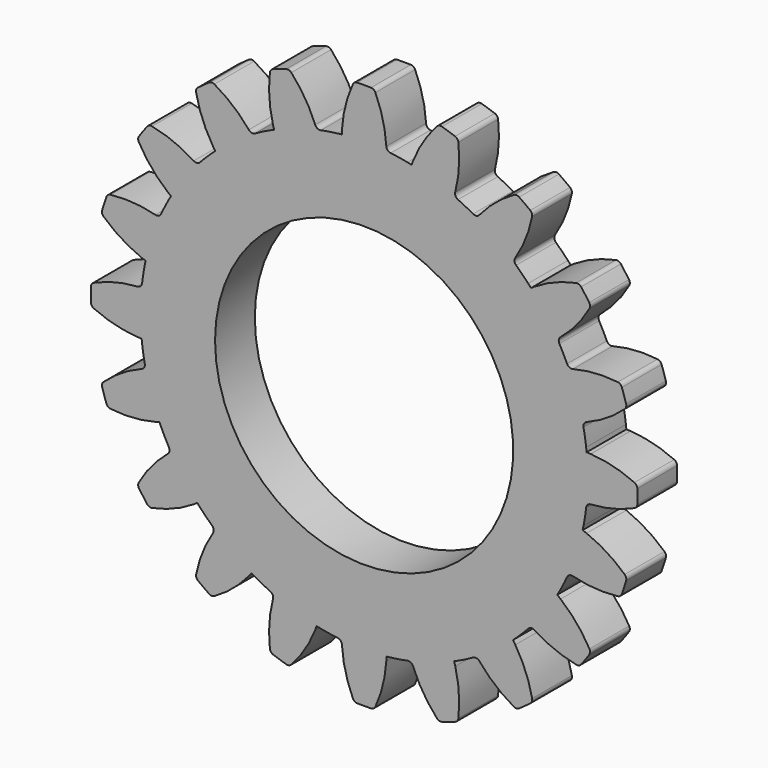
from build123d import *

# Parameters (mm, degrees)
F1_DEPTH    = 2
F2_COUNT    = 20
F4_T1_DEPTH = 2
F5_T1_DEPTH = 2
F7_D        = 12


# Not quite as in the source:
# - a fillet or chamfer that OpenCascade refuses, or shapes differently, is made with other operations: its cross-section is extruded or revolved along the edge and cut away or added


with BuildPart() as f1:
    # F0 (on Front) → F1 (new body)
    with BuildSketch(Plane.XZ):
        with BuildLine():
            Line((1.9112613806, 8.7947188662), (1.7449632612, 8.8292187206))
            ThreePointArc((1.7449632612, 8.8292187206), (1.4079101854, 8.8891950654), (1.0688199514, 8.9363093003))
            ThreePointArc((1.0688199514, 8.9363093003), (0.946985122, 8.9977640685), (0.8929222618, 9.1230542171))
            ThreePointArc((0.8929222618, 9.1230542171), (0.7550782147, 10.0220561804), (0.4535111269, 10.880113756))
            ThreePointArc((0.4535111269, 10.880113756), (0.3818211789, 10.9635928884), (0.2768246504, 10.9965161807))
            ThreePointArc((0.2768246504, 10.9965161807), (0, 11), (-0.2768246504, 10.9965161807))
            ThreePointArc((-0.2768246504, 10.9965161807), (-0.3818211789, 10.9635928884), (-0.4535111269, 10.880113756))
            ThreePointArc((-0.4535111269, 10.880113756), (-0.7550782147, 10.0220561804), (-0.8929222618, 9.1230542171))
            Line((-0.8929222618, 9.1230542171), (-0.9, 8.954886934))
            Line((-0.9, 8.954886934), (0, 0))
            Line((0, 0), (1.9112613806, 8.7947188662))
        make_face()
    extrude(amount=F1_DEPTH)


with BuildPart() as f2_1:
    # F2: instance of F1
    add(f1.part.rotate(Axis((0, -1, 0), (0, 1, 0)), 1 * 360 / F2_COUNT))


with BuildPart() as f2_2:
    # F2: instance of F1
    add(f1.part.rotate(Axis((0, -1, 0), (0, 1, 0)), 2 * 360 / F2_COUNT))


with BuildPart() as f2_3:
    # F2: instance of F1
    add(f1.part.rotate(Axis((0, -1, 0), (0, 1, 0)), 3 * 360 / F2_COUNT))


with BuildPart() as f2_4:
    # F2: instance of F1
    add(f1.part.rotate(Axis((0, -1, 0), (0, 1, 0)), 4 * 360 / F2_COUNT))


with BuildPart() as f2_5:
    # F2: instance of F1
    add(f1.part.rotate(Axis((0, -1, 0), (0, 1, 0)), 5 * 360 / F2_COUNT))


with BuildPart() as f2_6:
    # F2: instance of F1
    add(f1.part.rotate(Axis((0, -1, 0), (0, 1, 0)), 6 * 360 / F2_COUNT))


with BuildPart() as f2_7:
    # F2: instance of F1
    add(f1.part.rotate(Axis((0, -1, 0), (0, 1, 0)), 7 * 360 / F2_COUNT))


with BuildPart() as f2_8:
    # F2: instance of F1
    add(f1.part.rotate(Axis((0, -1, 0), (0, 1, 0)), 8 * 360 / F2_COUNT))


with BuildPart() as f2_9:
    # F2: instance of F1
    add(f1.part.rotate(Axis((0, -1, 0), (0, 1, 0)), 9 * 360 / F2_COUNT))


with BuildPart() as f2_10:
    # F2: instance of F1
    add(f1.part.rotate(Axis((0, -1, 0), (0, 1, 0)), 10 * 360 / F2_COUNT))


with BuildPart() as f2_11:
    # F2: instance of F1
    add(f1.part.rotate(Axis((0, -1, 0), (0, 1, 0)), 11 * 360 / F2_COUNT))


with BuildPart() as f2_12:
    # F2: instance of F1
    add(f1.part.rotate(Axis((0, -1, 0), (0, 1, 0)), 12 * 360 / F2_COUNT))


with BuildPart() as f2_13:
    # F2: instance of F1
    add(f1.part.rotate(Axis((0, -1, 0), (0, 1, 0)), 13 * 360 / F2_COUNT))


with BuildPart() as f2_14:
    # F2: instance of F1
    add(f1.part.rotate(Axis((0, -1, 0), (0, 1, 0)), 14 * 360 / F2_COUNT))


with BuildPart() as f2_15:
    # F2: instance of F1
    add(f1.part.rotate(Axis((0, -1, 0), (0, 1, 0)), 15 * 360 / F2_COUNT))


with BuildPart() as f2_16:
    # F2: instance of F1
    add(f1.part.rotate(Axis((0, -1, 0), (0, 1, 0)), 16 * 360 / F2_COUNT))


with BuildPart() as f2_17:
    # F2: instance of F1
    add(f1.part.rotate(Axis((0, -1, 0), (0, 1, 0)), 17 * 360 / F2_COUNT))


with BuildPart() as f2_18:
    # F2: instance of F1
    add(f1.part.rotate(Axis((0, -1, 0), (0, 1, 0)), 18 * 360 / F2_COUNT))


with BuildPart() as f2_19:
    # F2: instance of F1
    add(f1.part.rotate(Axis((0, -1, 0), (0, 1, 0)), 19 * 360 / F2_COUNT))


with BuildPart() as f2_1_1:
    add(f2_1.part)

    # F3: union F2_19, F2_18, F2_17, F2_16, F2_15, F2_14, F2_13, F2_12, F2_11, F2_10, F2_9, F2_8, F2_7, F2_6, F2_5, F2_4, F2_3, F2_2, F1
    add(f2_19.part)
    add(f2_18.part)
    add(f2_17.part)
    add(f2_16.part)
    add(f2_15.part)
    add(f2_14.part)
    add(f2_13.part)
    add(f2_12.part)
    add(f2_11.part)
    add(f2_10.part)
    add(f2_9.part)
    add(f2_8.part)
    add(f2_7.part)
    add(f2_6.part)
    add(f2_5.part)
    add(f2_4.part)
    add(f2_3.part)
    add(f2_2.part)
    add(f1.part)

    # F4: fillet of radius 0.2 on 1 edges, made by hand

    # F4_s2 → F4_t1 (join)
    with BuildSketch(Plane.XZ):
        with BuildLine():
            ThreePointArc((8.4039239655, 3.6693224205), (8.2654440862, 3.6807989412), (8.1678639962, 3.7797257501))
            Line((8.1678639962, 3.7797257501), (8.2384882763, 3.62316311))
            Line((8.2384882763, 3.62316311), (8.4039239655, 3.6693224205))
        make_face()
    extrude(amount=F4_T1_DEPTH)

    # F5: fillet of radius 0.2 on 1 edges, made by hand

    # F5_s2 → F5_t1 (join)
    with BuildSketch(Plane.XZ):
        with BuildLine():
            ThreePointArc((4.6421437029, 7.9082467644), (4.5233653976, 7.8361350338), (4.3862737271, 7.8588123656))
            Line((4.3862737271, 7.8588123656), (4.5354351808, 7.7736624393))
            Line((4.5354351808, 7.7736624393), (4.6421437029, 7.9082467644))
        make_face()
    extrude(amount=F5_T1_DEPTH)

    # F7 (through all)
    with Locations(Plane.XZ.offset(2)):
        with Locations((0, 0)):
            Hole(F7_D / 2)


solid = f2_1_1.part
